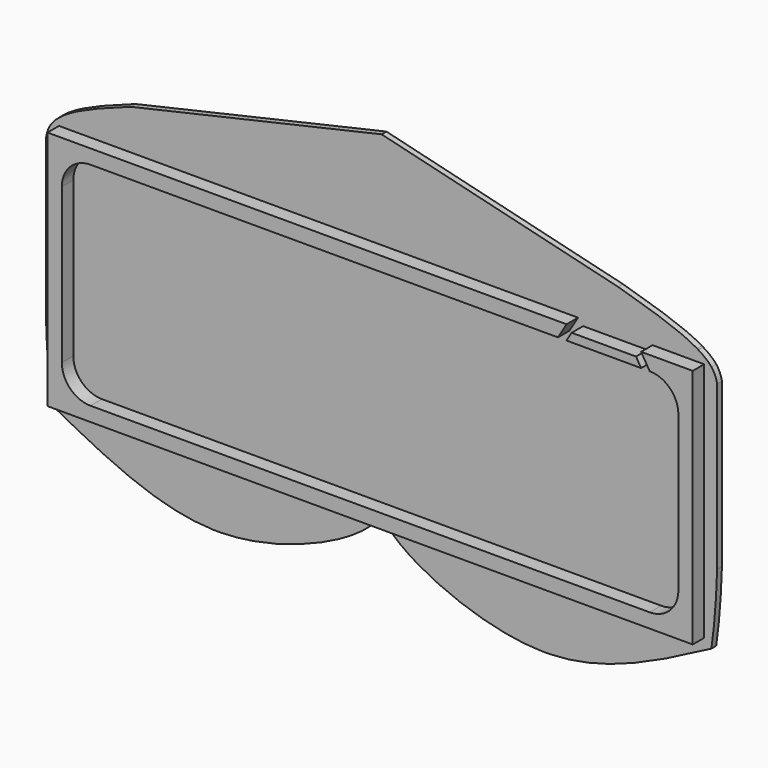
from build123d import *

# Parameters (mm, degrees)
F0_W     = 584.2
F0_H     = 219.71
F1_DEPTH = 5.334
F2_W     = 571.5
F2_H     = 213.36
F2_W_2   = 546.1
F2_H_2   = 187.96
F3_DEPTH = 12.7
F4_R     = 25.4
F6_DEPTH = 12.7
F8_DEPTH = 5.334
F9_DEPTH = 5.334


# Not quite as in the source:
# - a feature names something its author has since deleted; it is built from what else it names


with BuildPart() as f1:
    # F0 (on Front) → F1 (new body)
    with BuildSketch(Plane.XZ):
        with Locations((-292.1, 109.855)):
            Rectangle(F0_W, F0_H)
    extrude(amount=F1_DEPTH)

    # F2 (on face) → F3 (join)
    with BuildSketch(Plane.XZ.offset(5.334)):
        with Locations((-292.1, 113.03)):
            Rectangle(F2_W, F2_H)
        with Locations((-292.1, 113.03)):
            Rectangle(F2_W_2, F2_H_2, mode=Mode.SUBTRACT)
    extrude(amount=F3_DEPTH)

    # F4
    f4_edges = [f1.edges().sort_by_distance(p)[0] for p in [
        (-565.15, -11.684, 207.01),
        (-19.05, -11.684, 207.01),
        (-19.05, -11.684, 19.05),
        (-565.15, -11.684, 19.05),
    ]]
    fillet(f4_edges, radius=F4_R)

    # F5 (on face) → F6 (cut)
    with BuildSketch(Plane.XZ.offset(18.034)):
        Polygon((-118.11, 219.71), (-125.73, 207.01), (-118.11, 207.01), (-113.5820166854, 214.5566388576), (-110.49, 219.71), align=None)
        Polygon((-56.5979833146, 214.5566388576), (-52.07, 207.01), (-44.45, 207.01), (-52.07, 219.71), (-59.69, 219.71), align=None)
        Polygon((-59.69, 219.71), (-110.49, 219.71), (-113.5820166854, 214.5566388576), (-56.5979833146, 214.5566388576), align=None)
    extrude(amount=-F6_DEPTH, mode=Mode.SUBTRACT)

    # F7 (on face) → F8 (cut)
    with BuildSketch(Plane(origin=(0, 0, 0), x_dir=(-1, 0, 0), z_dir=(0, 1, 0))):
        with BuildLine():
            add(Edge.make_bspline(
                [(292.1, 6.35), (289.8878914708, 4.2388101088), (287.6757829415, 2.1276202176), (285.3383261504, 0)],
                knots=[0, 0, 0, 0, 0.0566650496, 0.0566650496, 0.0566650496, 0.0566650496], degree=3))
            Line((285.3383261504, 0), (292.1, 0))
            Line((292.1, 0), (292.1, 6.35))
        make_face()
        with BuildLine():
            add(Edge.make_bspline(
                [(292.1, 6.35), (294.3115112442, 4.2388053382), (296.5230224884, 2.1276106765), (298.8599853109, 0)],
                knots=[0, 0, 0, 0, 0.056662645, 0.056662645, 0.056662645, 0.056662645], degree=3))
            Line((292.1, 6.35), (292.1, 0))
            Line((292.1, 0), (298.8599853109, 0))
        make_face()
    extrude(amount=-F8_DEPTH, mode=Mode.SUBTRACT)

    # F7 (on face) → F9 (join)
    with BuildSketch(Plane(origin=(0, 0, 0), x_dir=(-1, 0, 0), z_dir=(0, 1, 0))):
        with BuildLine():
            Line((285.3383261504, 0), (0, 0))
            add(Edge.make_bspline(
                [(35.5548654074, -18.4164866805), (23.6750755263, -12.5314961521), (11.8375377632, -6.265748076), (0, 0)],
                knots=[0.8952858021, 0.8952858021, 0.8952858021, 0.8952858021, 1, 1, 1, 1], degree=3))
            Line((35.5548654074, -18.4164866805), (260.35, -18.4164866805))
            add(Edge.make_bspline(
                [(285.3383261504, 0), (278.8607301271, -5.8960937002), (271.4205053001, -11.9183662972), (260.35, -18.4164866805)],
                knots=[0.0566650496, 0.0566650496, 0.0566650496, 0.0566650496, 0.2136961022, 0.2136961022, 0.2136961022, 0.2136961022], degree=3))
        make_face()
        with BuildLine():
            add(Edge.make_bspline(
                [(0, 0), (-2.7059325948, 17.274832353), (-4.5181928473, 42.574440276), (-5.08, 63.5)],
                knots=[0, 0, 0, 0, 0.5267133936, 0.5267133936, 0.5267133936, 0.5267133936], degree=3))
            Line((0, 0), (0, 219.71))
            add(Edge.make_bspline(
                [(0, 219.71), (-2.907575848, 216.0546733014), (-4.393729889, 212.1257933571), (-5.08, 208.0429754021)],
                knots=[0.6401685719, 0.6401685719, 0.6401685719, 0.6401685719, 0.7975102285, 0.7975102285, 0.7975102285, 0.7975102285], degree=3))
            Line((-5.08, 208.0429754021), (-5.08, 191.77))
            Line((-5.08, 191.77), (-5.08, 114.935))
            Line((-5.08, 114.935), (-5.08, 63.5))
        make_face()
        with BuildLine():
            Line((260.35, -18.4164866805), (35.5548654074, -18.4164866805))
            add(Edge.make_bspline(
                [(143.5928555626, -50.8), (106.470496214, -50.0055886792), (70.8264502644, -35.8892656507), (35.5548654074, -18.4164866805)],
                knots=[0.5843850409, 0.5843850409, 0.5843850409, 0.5843850409, 0.8952858021, 0.8952858021, 0.8952858021, 0.8952858021], degree=3))
            Line((143.5928555626, -50.8), (150.3785817486, -50.8))
            add(Edge.make_bspline(
                [(260.35, -18.4164866805), (235.5497171967, -32.973656279), (192.5306851802, -49.9188924594), (150.3785817486, -50.8)],
                knots=[0.2136961022, 0.2136961022, 0.2136961022, 0.2136961022, 0.5654790071, 0.5654790071, 0.5654790071, 0.5654790071], degree=3))
        make_face()
        with BuildLine():
            add(Edge.make_bspline(
                [(11.5967126237, 229.2998559787), (6.6790583406, 226.3057112292), (2.7183257178, 223.1274064895), (0, 219.71)],
                knots=[0.4930680682, 0.4930680682, 0.4930680682, 0.4930680682, 0.6401685719, 0.6401685719, 0.6401685719, 0.6401685719], degree=3))
            Line((0, 219.71), (292.1, 219.71))
            Line((292.1, 219.71), (11.5967126237, 229.2998559787))
        make_face()
        with BuildLine():
            add(Edge.make_bspline(
                [(12.5483744012, 229.87), (12.2273175537, 229.6806902818), (11.9100723395, 229.4906470132), (11.5967126237, 229.2998559787)],
                knots=[0.4836946212, 0.4836946212, 0.4836946212, 0.4836946212, 0.4930680682, 0.4930680682, 0.4930680682, 0.4930680682], degree=3))
            Line((11.5967126237, 229.2998559787), (292.1, 219.71))
            Line((292.1, 219.71), (573.5876283802, 229.3335086626))
            add(Edge.make_bspline(
                [(572.7896932404, 229.87), (573.0585490403, 229.6916783135), (573.3245454934, 229.5128510633), (573.5876283802, 229.3335086626)],
                knots=[0.4655830842, 0.4655830842, 0.4655830842, 0.4655830842, 0.4744116019, 0.4744116019, 0.4744116019, 0.4744116019], degree=3))
            Line((572.7896932404, 229.87), (514.35, 229.87))
            Line((514.35, 229.87), (292.1, 229.87))
            Line((292.1, 229.87), (82.55, 229.87))
            Line((82.55, 229.87), (12.5483744012, 229.87))
        make_face()
        with BuildLine():
            Line((573.5876283802, 229.3335086626), (292.1, 219.71))
            Line((292.1, 219.71), (584.2, 219.71))
            add(Edge.make_bspline(
                [(573.5876283802, 229.3335086626), (578.0527057549, 226.2896858373), (581.6785208511, 223.0974722581), (584.2, 219.71)],
                knots=[0.4744116019, 0.4744116019, 0.4744116019, 0.4744116019, 0.6242503674, 0.6242503674, 0.6242503674, 0.6242503674], degree=3))
        make_face()
        with BuildLine():
            add(Edge.make_bspline(
                [(298.8599853109, 0), (305.3364495341, -5.8962831133), (312.7764065366, -11.9186444461), (323.85, -18.4164866805)],
                knots=[0.056662645, 0.056662645, 0.056662645, 0.056662645, 0.2136927825, 0.2136927825, 0.2136927825, 0.2136927825], degree=3))
            Line((323.85, -18.4164866805), (548.6673215949, -18.4164866805))
            add(Edge.make_bspline(
                [(548.6673215949, -18.4164866805), (560.540064076, -12.5314899408), (572.370032038, -6.2657449704), (584.2, 0)],
                knots=[0.8952964295, 0.8952964295, 0.8952964295, 0.8952964295, 1, 1, 1, 1], degree=3))
            Line((584.2, 0), (298.8599853109, 0))
        make_face()
        with BuildLine():
            Line((548.6673215949, -18.4164866805), (323.85, -18.4164866805))
            add(Edge.make_bspline(
                [(323.85, -18.4164866805), (348.6543054028, -32.9713340996), (391.6899454814, -49.9118498543), (433.8458201185, -50.8)],
                knots=[0.2136927825, 0.2136927825, 0.2136927825, 0.2136927825, 0.5654325768, 0.5654325768, 0.5654325768, 0.5654325768], degree=3))
            Line((433.8458201185, -50.8), (440.69, -50.8))
            add(Edge.make_bspline(
                [(440.69, -50.8), (477.8051745876, -49.9992725657), (513.4246952416, -35.8853016167), (548.6673215949, -18.4164866805)],
                knots=[0.5844980763, 0.5844980763, 0.5844980763, 0.5844980763, 0.8952964295, 0.8952964295, 0.8952964295, 0.8952964295], degree=3))
        make_face()
        with BuildLine():
            add(Edge.make_bspline(
                [(82.55, 255.27), (55.8328777889, 247.4544406939), (29.1157555777, 239.6388813877), (12.5483744012, 229.87)],
                knots=[0, 0, 0, 0, 0.4836946212, 0.4836946212, 0.4836946212, 0.4836946212], degree=3))
            Line((12.5483744012, 229.87), (82.55, 229.87))
            Line((82.55, 229.87), (82.55, 255.27))
        make_face()
        with BuildLine():
            add(Edge.make_bspline(
                [(584.2, 219.71), (587.2466521414, 215.6169859397), (588.681040168, 211.2389059428), (589.28, 206.7131131)],
                knots=[0.6242503674, 0.6242503674, 0.6242503674, 0.6242503674, 0.8052975103, 0.8052975103, 0.8052975103, 0.8052975103], degree=3))
            Line((584.2, 219.71), (584.2, 0))
            add(Edge.make_bspline(
                [(584.2, 0), (587.0231389999, 19.4493960589), (588.7459289581, 43.301401327), (589.28, 63.5)],
                knots=[0, 0, 0, 0, 0.5267133936, 0.5267133936, 0.5267133936, 0.5267133936], degree=3))
            Line((589.28, 63.5), (589.28, 114.935))
            Line((589.28, 114.935), (589.28, 191.77))
            Line((589.28, 191.77), (589.28, 206.7131131))
        make_face()
        with BuildLine():
            Line((82.55, 255.27), (82.55, 229.87))
            Line((82.55, 229.87), (292.1, 229.87))
            Line((292.1, 229.87), (292.1, 306.07))
            add(Edge.make_bspline(
                [(292.1, 306.07), (222.25, 289.1366666667), (152.4, 272.2033333333), (82.55, 255.27)],
                knots=[0, 0, 0, 0, 215.6196709486, 215.6196709486, 215.6196709486, 215.6196709486], degree=3))
        make_face()
        with BuildLine():
            Line((514.35, 229.87), (572.7896932404, 229.87))
            add(Edge.make_bspline(
                [(514.35, 255.27), (536.4806207919, 247.2720101715), (558.6112415838, 239.274020343), (572.7896932404, 229.87)],
                knots=[0, 0, 0, 0, 0.4655830842, 0.4655830842, 0.4655830842, 0.4655830842], degree=3))
            Line((514.35, 255.27), (514.35, 229.87))
        make_face()
        with BuildLine():
            Line((292.1, 306.07), (292.1, 229.87))
            Line((292.1, 229.87), (514.35, 229.87))
            Line((514.35, 229.87), (514.35, 255.27))
            add(Edge.make_bspline(
                [(514.35, 255.27), (440.2666666667, 272.2033333333), (366.1833333333, 289.1366666667), (292.1, 306.07)],
                knots=[0, 0, 0, 0, 227.9818030019, 227.9818030019, 227.9818030019, 227.9818030019], degree=3))
        make_face()
    extrude(amount=-F9_DEPTH)


solid = f1.part
